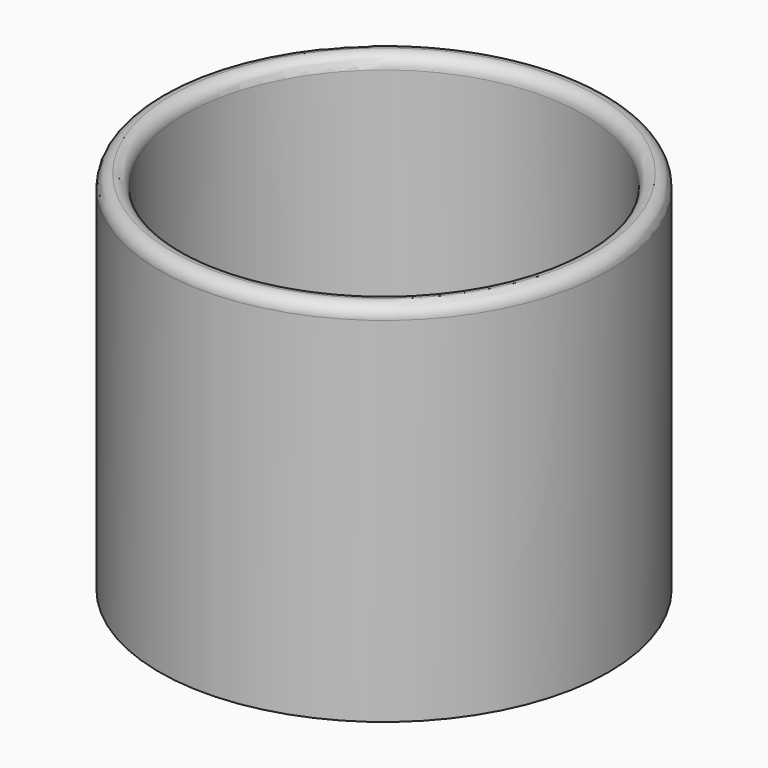
from build123d import *

# Parameters (mm, degrees)
F1_R = 22.4423927589
F3_T = -2.54
F4_R = 1.26999


# Not quite as in the source:
# - a fillet or chamfer is up to 0.001 mm smaller than in the source, because OpenCascade refuses the exact size


with BuildPart() as f2:
    # F2: sweep along a path in F0
    with BuildLine(Plane.XZ) as f2_path:
        Line((-22.9121223092, 36.5854799747), (-22.9121223092, 0))
    # F1 (on Top) → F2 (sweep)
    with BuildSketch(Plane.XY):
        Circle(F1_R)
    sweep(path=f2_path.line)

    # F3
    f3_openings = [f2.faces().sort_by_distance(p)[0] for p in [
        (0, 0, 36.58548),
    ]]
    offset(amount=F3_T, openings=f3_openings)

    # F4 (radius 1.27 in the source; OpenCascade refuses exactly that, so slightly less here)
    f4_edges = [f2.edges().sort_by_distance(p)[0] for p in [
        (-22.442393, 0, 36.58548),
        (-19.902393, 0, 36.58548),
    ]]
    fillet(f4_edges, radius=F4_R)


solid = f2.part
